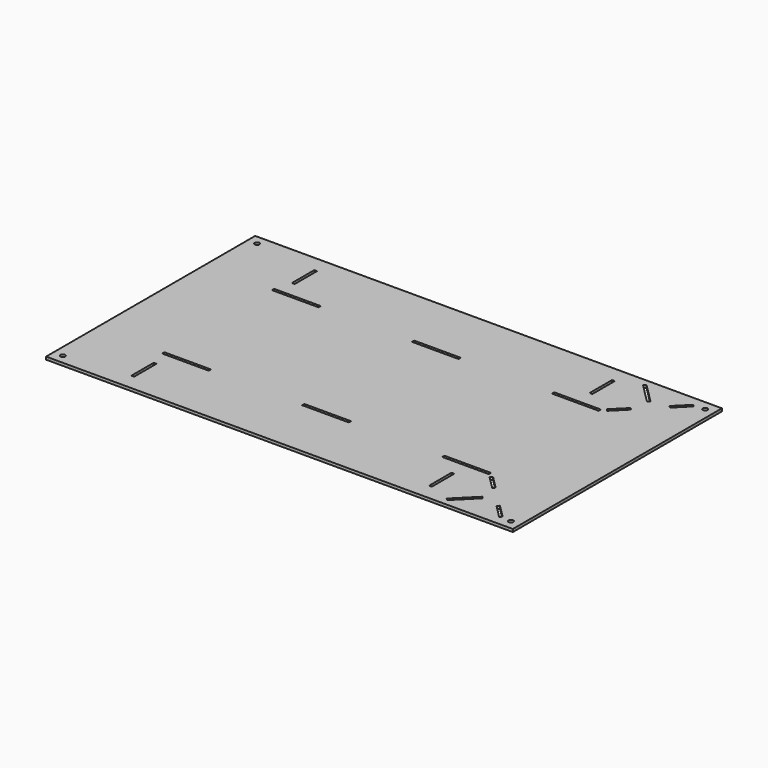
from build123d import *

# Parameters (mm, degrees)
F0_W     = 2.95
F0_H     = 30
F0_W_2   = 50
F0_H_2   = 2.95
F1_DEPTH = 2.95
F3_D     = 5
F5_DEPTH = 2.95


# Not quite as in the source:
# - a feature names something its author has since deleted; it is built from what else it names


with BuildPart() as f1:
    # F0 (on Top) → F1 (new body)
    with BuildSketch(Plane.XY):
        Polygon((-37.9051826894, 0), (12.0948173106, 0), (462.0948173106, 0), (462.0948173106, 280), (62.0948173106, 280), (-37.9051826894, 280), align=None)
        with Locations((40.9065613726, 32.5)):
            Rectangle(F0_W, F0_H, mode=Mode.SUBTRACT)
        with Locations((59.4315613726, 66.475)):
            Rectangle(F0_W_2, F0_H_2, mode=Mode.SUBTRACT)
        with Locations((209.4315613726, 66.475)):
            Rectangle(F0_W_2, F0_H_2, mode=Mode.SUBTRACT)
        with Locations((359.8315613726, 32.5)):
            Rectangle(F0_W, F0_H, mode=Mode.SUBTRACT)
        with Locations((359.4315613726, 66.475)):
            Rectangle(F0_W_2, F0_H_2, mode=Mode.SUBTRACT)
        with Locations((59.4315613726, 213.525)):
            Rectangle(F0_W_2, F0_H_2, mode=Mode.SUBTRACT)
        with Locations((40.9065613726, 247.5)):
            Rectangle(F0_W, F0_H, mode=Mode.SUBTRACT)
        with Locations((209.4315613726, 213.525)):
            Rectangle(F0_W_2, F0_H_2, mode=Mode.SUBTRACT)
        with Locations((359.4315613726, 213.525)):
            Rectangle(F0_W_2, F0_H_2, mode=Mode.SUBTRACT)
        with Locations((359.8315613726, 247.5)):
            Rectangle(F0_W, F0_H, mode=Mode.SUBTRACT)
    extrude(amount=F1_DEPTH)

    # F3 (through all)
    with Locations(Plane.XY.offset(2.95)):
        with Locations((-27.9051826894, 10), (-27.9051826894, 270), (452.0948173106, 10), (452.0948173106, 270)):
            Hole(F3_D / 2)

    # F4 (on face) → F5 (cut)
    with BuildSketch(Plane.XY.offset(2.95)):
        Polygon((402.1092280247, 232.6776666521), (387.9670924009, 218.5355310284), (390.0530574054, 216.4495660239), (404.1951930292, 230.5917016476), align=None)
        Polygon((441.5175263771, 267.9140349955), (439.4315613726, 270), (425.2894257488, 255.8578643763), (427.3753907533, 253.7718993718), align=None)
        Polygon((386.4580381415, 273.5950192639), (384.372073137, 271.5090542594), (405.5852765726, 250.2958508238), (407.6712415771, 252.3818158283), align=None)
        Polygon((386.4580381415, 6.4049807361), (407.6712415771, 27.6181841717), (405.5852765726, 29.7041491762), (384.372073137, 8.4909457406), align=None)
        Polygon((427.3753907533, 26.2281006282), (425.2894257488, 24.1421356237), (439.4315613726, 10), (441.5175263771, 12.0859650045), align=None)
        Polygon((387.9670924009, 61.4644689716), (402.1092280247, 47.3223333479), (404.1951930292, 49.4082983524), (390.0530574054, 63.5504339761), align=None)
    extrude(amount=-F5_DEPTH, mode=Mode.SUBTRACT)


solid = f1.part
